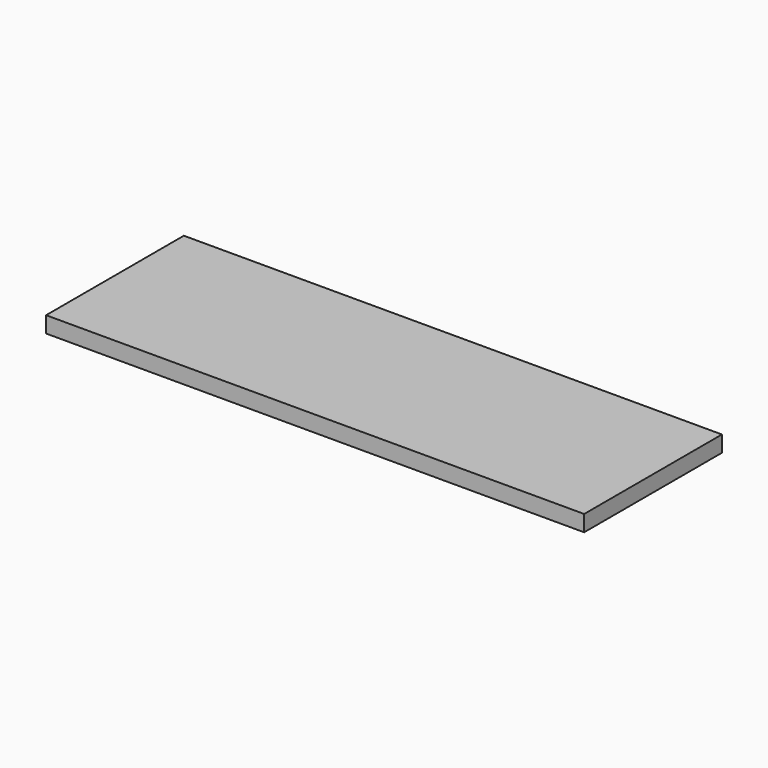
from build123d import *

# Parameters (mm, degrees)
F0_W     = 317.5
F0_H     = 101.6
F1_DEPTH = 9.525


# Not quite as in the source:
# - a length typed as a fraction of an inch, garbled in the dataset ("3 / 203.2 mm" for 3/8 in), is restored


with BuildPart() as f1:
    # F0 (on Top) → F1 (new body)
    with BuildSketch(Plane.XY):
        Rectangle(F0_W, F0_H)
    extrude(amount=F1_DEPTH)


solid = f1.part
